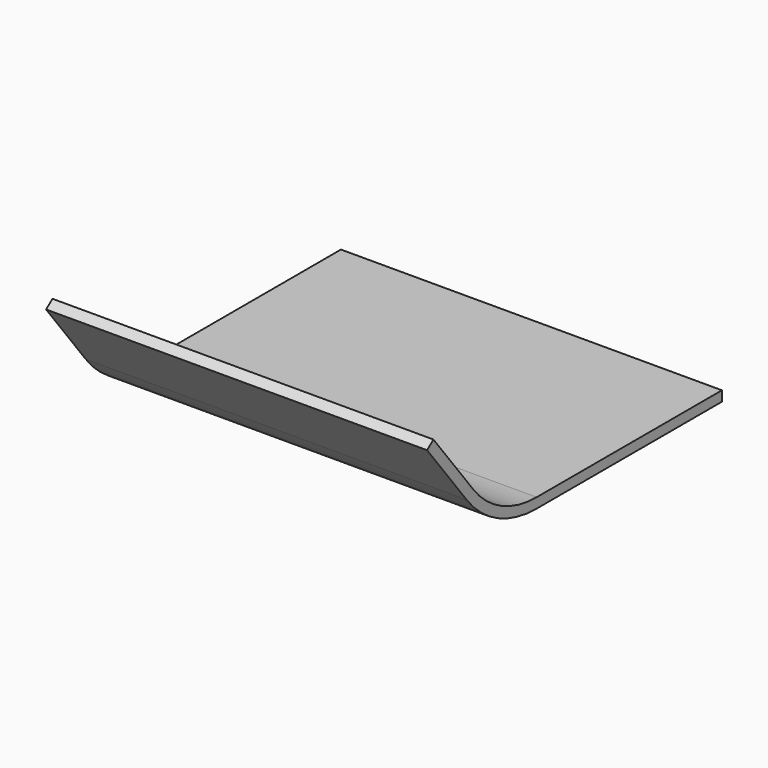
from build123d import *

# Parameters (mm, degrees)
F1_DEPTH = 416


# Not quite as in the source:
# - ends of sketch curves that miss each other by under 0.0002 mm in the source are joined


with BuildPart() as f1:
    # F0 (on Right) → F1 (new body)
    with BuildSketch(Plane.YZ):
        with BuildLine():
            Line((201.222667, -50.876591), (-51.671206, -50.876591))
            ThreePointArc((-51.671206, -50.876591), (-99.9341457634, -39.609331908), (-138.2192681533, -8.1369331174))
            Line((-138.2192681533, -8.1369331174), (-192.531195, 61.87659))
            Line((-192.531195, 61.87659), (-201.222667, 55.134312))
            Line((-201.222667, 55.134312), (-146.931681, -14.852216))
            ThreePointArc((-146.931681, -14.852216), (-104.7886465547, -49.480203899), (-51.671206, -61.876591))
            Line((-51.671206, -61.876591), (201.222667, -61.876591))
            Line((201.222667, -61.876591), (201.222667, -50.876591))
        make_face()
    extrude(amount=F1_DEPTH)


solid = f1.part
